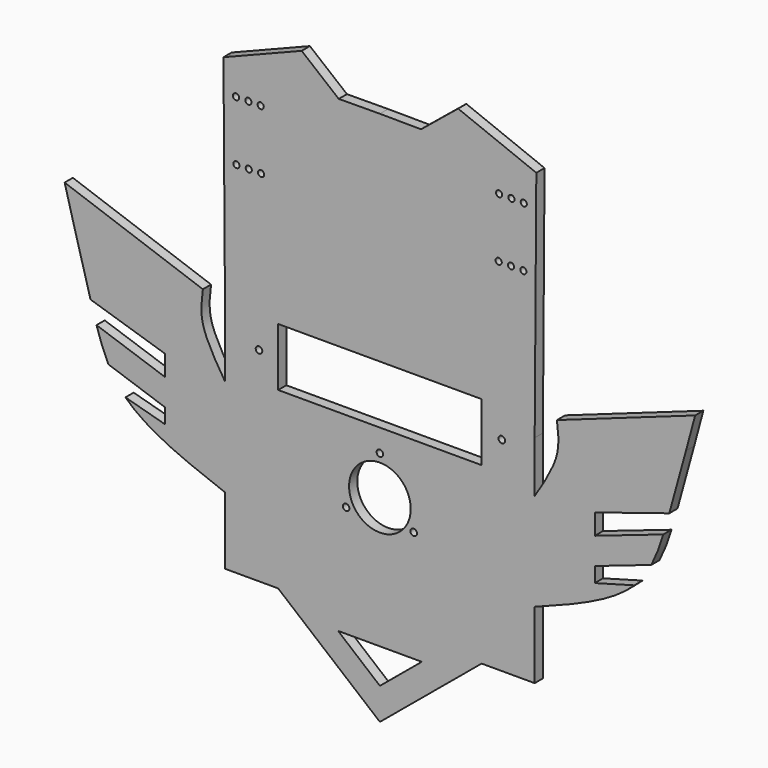
from build123d import *

# Parameters (mm, degrees)
F0_R     = 1.6
F0_R_2   = 15
F0_R_3   = 1.5
F1_DEPTH = 5


# Not quite as in the source:
# - ends of sketch curves that miss each other by under 0.0002 mm in the source are joined


with BuildPart() as f1:
    # F0 (on Front) → F1 (new body)
    with BuildSketch(Plane.XZ):
        Polygon((-96.9045388699, -40.5384600163), (-146.4045388699, -40.5384600163), (-96.9045388699, -81.6254615784), (-47.4045388699, -40.5384600163), align=None)
        Polygon((-96.9045388699, -66.1772739545), (-117.2328144312, -49.2524243891), (-76.514147222, -49.2524243891), align=None, mode=Mode.SUBTRACT)
        Polygon((-116.9301321116, 178.7101170527), (-173.0099775762, 178.315364934), (-172.209293991, 64.5674973527), (-172.209293991, 39.6003018865), (-172.209293991, -7.8263543546), (-172.209293991, -40.5384600163), (-146.4045388699, -40.5384600163), (-96.9045388699, -40.5384600163), (-47.4045388699, -40.5384600163), (-21.5997837488, -40.5384600163), (-21.5997837488, -7.8263543546), (-21.5997837488, 39.6003018865), (-21.5997837488, 64.5674973527), (-20.7991001636, 178.315364934), (-76.8789456281, 178.7101170527), (-96.9045388699, 178.851079377), align=None)
        with Locations((-113.3590215418, 4.9431557872)):
            Circle(F0_R, mode=Mode.SUBTRACT)
        with Locations((-96.9045388699, 14.4431557872)):
            Circle(F0_R_2, mode=Mode.SUBTRACT)
        with Locations((-96.9045388699, 33.4431557872)):
            Circle(F0_R, mode=Mode.SUBTRACT)
        with Locations((-80.450056198, 4.9431557872)):
            Circle(F0_R, mode=Mode.SUBTRACT)
        with Locations((-166.7004097796, 134.3582146961)):
            Circle(F0_R_3, mode=Mode.SUBTRACT)
        with Locations((-160.7005600937, 134.4006852416)):
            Circle(F0_R_3, mode=Mode.SUBTRACT)
        with Locations((-154.7007104079, 134.4431557872)):
            Circle(F0_R_3, mode=Mode.SUBTRACT)
        with Locations((-166.9045388699, 163.3574962616)):
            Circle(F0_R_3, mode=Mode.SUBTRACT)
        with Locations((-160.904689184, 163.3999668071)):
            Circle(F0_R_3, mode=Mode.SUBTRACT)
        with Locations((-154.9048394982, 163.4424373527)):
            Circle(F0_R_3, mode=Mode.SUBTRACT)
        Polygon((-160.5466744936, 58.5852914109), (-146.4045388699, 72.7274270346), (-47.4045388699, 72.7274270346), (-33.2624032461, 58.5852914109), (-47.4045388699, 44.4431557872), (-146.4045388699, 44.4431557872), align=None, mode=Mode.SUBTRACT)
        with Locations((-39.1083673318, 134.4431557872)):
            Circle(F0_R_3, mode=Mode.SUBTRACT)
        with Locations((-33.108517646, 134.4006852416)):
            Circle(F0_R_3, mode=Mode.SUBTRACT)
        with Locations((-27.1086679602, 134.3582146961)):
            Circle(F0_R_3, mode=Mode.SUBTRACT)
        with Locations((-38.9042382416, 163.4424373527)):
            Circle(F0_R_3, mode=Mode.SUBTRACT)
        with Locations((-32.9043885557, 163.3999668071)):
            Circle(F0_R_3, mode=Mode.SUBTRACT)
        with Locations((-26.9045388699, 163.3574962616)):
            Circle(F0_R_3, mode=Mode.SUBTRACT)
        with BuildLine():
            add(Edge.make_bspline(
                [(-10.7653314617, 75.6704937657), (-10.1423011883, 70.9060238986), (-8.7253114516, 60.0699454768), (-16.9765192292, 46.9510213145), (-21.5997880701, 39.6003018865)],
                knots=[0, 0, 0, 0, 0.4396858053, 1, 1, 1, 1], degree=3))
            Line((-21.5997880701, 39.6003018865), (-21.5997837488, -7.8263543546))
            add(Edge.make_bspline(
                [(26.8901133537, 17.1408411115), (16.0887779237, 6.4091763607), (-2.7555050732, -0.708588997), (-21.5997837488, -7.8263543546)],
                knots=[0.6427998281, 0.6427998281, 0.6427998281, 0.6427998281, 1, 1, 1, 1], degree=3))
            Line((26.8901133537, 17.1408411115), (7.6417172557, 11.8470894728))
            Line((7.6417172557, 11.8470894728), (7.6417172557, 19.1424891602))
            Line((7.6417172557, 19.1424891602), (35.1491589972, 28.5522722191))
            add(Edge.make_bspline(
                [(40.9662291467, 43.4994469848), (39.3215463775, 38.1621436215), (37.5379634129, 33.1572861433), (35.1491589972, 28.5522722191)],
                knots=[0.4005507879, 0.4005507879, 0.4005507879, 0.4005507879, 0.528058188, 0.528058188, 0.528058188, 0.528058188], degree=3))
            Line((40.9662291467, 43.4994469848), (7.6417172557, 32.0997526626))
            Line((7.6417172557, 32.0997526626), (7.6417172557, 42.0997526626))
            Line((7.6417172557, 42.0997526626), (43.8890115662, 53.5073665746))
            add(Edge.make_bspline(
                [(52.0098697503, 82.9429342223), (49.2436269652, 72.7066022993), (46.514808756, 62.7382046066), (43.8890115662, 53.5073665746)],
                knots=[0.1175634385, 0.1175634385, 0.1175634385, 0.1175634385, 0.3236243824, 0.3236243824, 0.3236243824, 0.3236243824], degree=3))
            add(Edge.make_bspline(
                [(56.4675719729, 99.5147182414), (54.9776571845, 93.9620524152), (53.4884176136, 88.4142206812), (52.0098697503, 82.9429342223)],
                knots=[0.0074245274, 0.0074245274, 0.0074245274, 0.0074245274, 0.1175634385, 0.1175634385, 0.1175634385, 0.1175634385], degree=3))
            Line((56.4675719729, 99.5147182414), (-10.7653314617, 75.6704937657))
        make_face()
        with BuildLine():
            Line((-172.209293991, -7.8263543546), (-172.209293991, 39.6003018865))
            add(Edge.make_bspline(
                [(-183.043746278, 75.6704937657), (-183.6667765514, 70.9060238986), (-185.0837662881, 60.0699454768), (-176.8325585105, 46.9510213145), (-172.209293991, 39.6003018865)],
                knots=[0, 0, 0, 0, 0.4396858053, 1, 1, 1, 1], degree=3))
            Line((-183.043746278, 75.6704937657), (-250.2766497126, 99.5147182414))
            add(Edge.make_bspline(
                [(-250.2766497126, 99.5147182414), (-248.7867349243, 93.9620524152), (-247.2974953533, 88.4142206812), (-245.81894749, 82.9429342223)],
                knots=[0.0074245274, 0.0074245274, 0.0074245274, 0.0074245274, 0.1175634385, 0.1175634385, 0.1175634385, 0.1175634385], degree=3))
            add(Edge.make_bspline(
                [(-245.81894749, 82.9429342223), (-243.0527047049, 72.7066022993), (-240.3238864957, 62.7382046066), (-237.6980893059, 53.5073665746)],
                knots=[0.1175634385, 0.1175634385, 0.1175634385, 0.1175634385, 0.3236243824, 0.3236243824, 0.3236243824, 0.3236243824], degree=3))
            Line((-237.6980893059, 53.5073665746), (-201.4507949954, 42.0997526626))
            Line((-201.4507949954, 42.0997526626), (-201.4507949954, 32.0997526626))
            Line((-201.4507949954, 32.0997526626), (-234.7753068864, 43.4994469848))
            add(Edge.make_bspline(
                [(-234.7753068864, 43.4994469848), (-233.1306241172, 38.1621436215), (-231.3470411526, 33.1572861433), (-228.9582367369, 28.5522722191)],
                knots=[0.4005507879, 0.4005507879, 0.4005507879, 0.4005507879, 0.528058188, 0.528058188, 0.528058188, 0.528058188], degree=3))
            Line((-228.9582367369, 28.5522722191), (-201.4507949954, 19.1424891602))
            Line((-201.4507949954, 19.1424891602), (-201.4507949954, 11.8470894728))
            Line((-201.4507949954, 11.8470894728), (-220.6991910934, 17.1408411115))
            add(Edge.make_bspline(
                [(-220.6991910934, 17.1408411115), (-209.8978556634, 6.4091763607), (-191.0535726665, -0.708588997), (-172.209293991, -7.8263543546)],
                knots=[0.6427998281, 0.6427998281, 0.6427998281, 0.6427998281, 1, 1, 1, 1], degree=3))
        make_face()
        Polygon((-146.4045388699, 44.4431557872), (-146.4045388699, 72.7274270346), (-160.5466744936, 58.5852914109), align=None)
        with Locations((-155.7186983824, 58.5852914109)):
            Circle(F0_R, mode=Mode.SUBTRACT)
        Polygon((-33.2624032461, 58.5852914109), (-47.4045388699, 72.7274270346), (-47.4045388699, 44.4431557872), align=None)
        with Locations((-37.5883497596, 58.5852914109)):
            Circle(F0_R, mode=Mode.SUBTRACT)
        Polygon((-134.957258223, 193.4304237366), (-173.0099775762, 178.315364934), (-116.9301321116, 178.7101170527), align=None)
        Polygon((-58.8518195167, 193.4304237366), (-76.8789456281, 178.7101170527), (-20.7991001636, 178.315364934), align=None)
    extrude(amount=F1_DEPTH)


solid = f1.part
